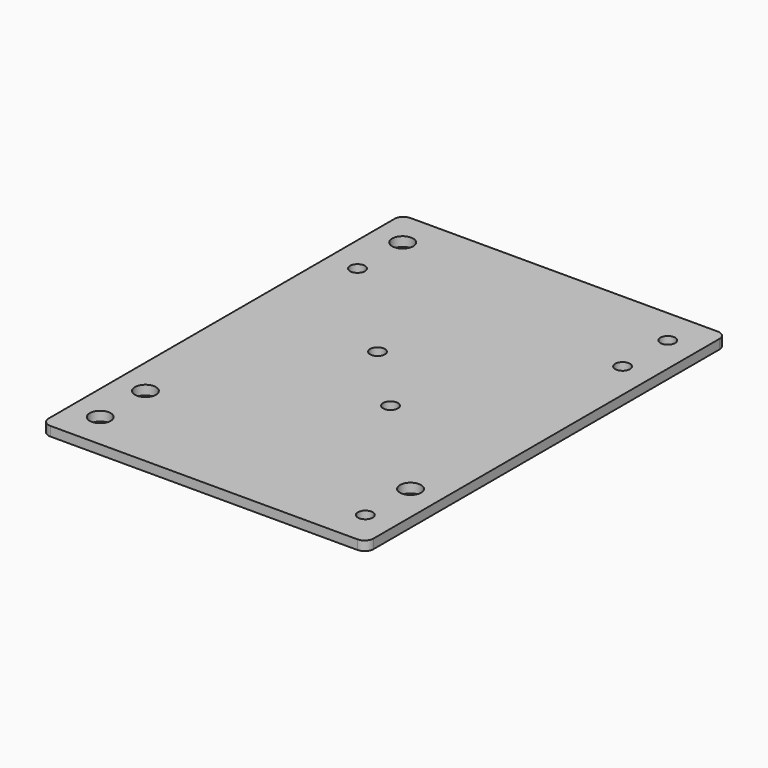
from build123d import *

# Parameters (mm, degrees)
F0_R     = 3.56
F0_R_2   = 2.5
F1_DEPTH = 3.175


# Not quite as in the source:
# - a length typed as a fraction of an inch, garbled in the dataset ("3 / 203.2 mm" for 3/8 in), is restored


with BuildPart() as f1:
    # F0 (on Top) → F1 (new body)
    with BuildSketch(Plane.XY):
        with BuildLine():
            ThreePointArc((55, 73.2), (54.1213203436, 75.3213203436), (52, 76.2))
            Line((52, 76.2), (-52, 76.2))
            ThreePointArc((-52, 76.2), (-54.1213203436, 75.3213203436), (-55, 73.2))
            Line((-55, 73.2), (-55, -73.2))
            ThreePointArc((-55, -73.2), (-54.1213203436, -75.3213203436), (-52, -76.2))
            Line((-52, -76.2), (52, -76.2))
            ThreePointArc((52, -76.2), (54.1213203436, -75.3213203436), (55, -73.2))
            Line((55, -73.2), (55, 73.2))
        make_face()
        with Locations((-44.875, -64)):
            Circle(F0_R, mode=Mode.SUBTRACT)
        with Locations((-44.875, -44.875)):
            Circle(F0_R, mode=Mode.SUBTRACT)
        with Locations((44.875, -64)):
            Circle(F0_R_2, mode=Mode.SUBTRACT)
        with Locations((44.875, -44.875)):
            Circle(F0_R, mode=Mode.SUBTRACT)
        with Locations((11, -11)):
            Circle(F0_R_2, mode=Mode.SUBTRACT)
        with Locations((-11, 11)):
            Circle(F0_R_2, mode=Mode.SUBTRACT)
        with Locations((-44.875, 44.875)):
            Circle(F0_R_2, mode=Mode.SUBTRACT)
        with Locations((-44.875, 64)):
            Circle(F0_R, mode=Mode.SUBTRACT)
        with Locations((44.875, 44.875)):
            Circle(F0_R_2, mode=Mode.SUBTRACT)
        with Locations((44.875, 64)):
            Circle(F0_R_2, mode=Mode.SUBTRACT)
    extrude(amount=F1_DEPTH)


solid = f1.part
